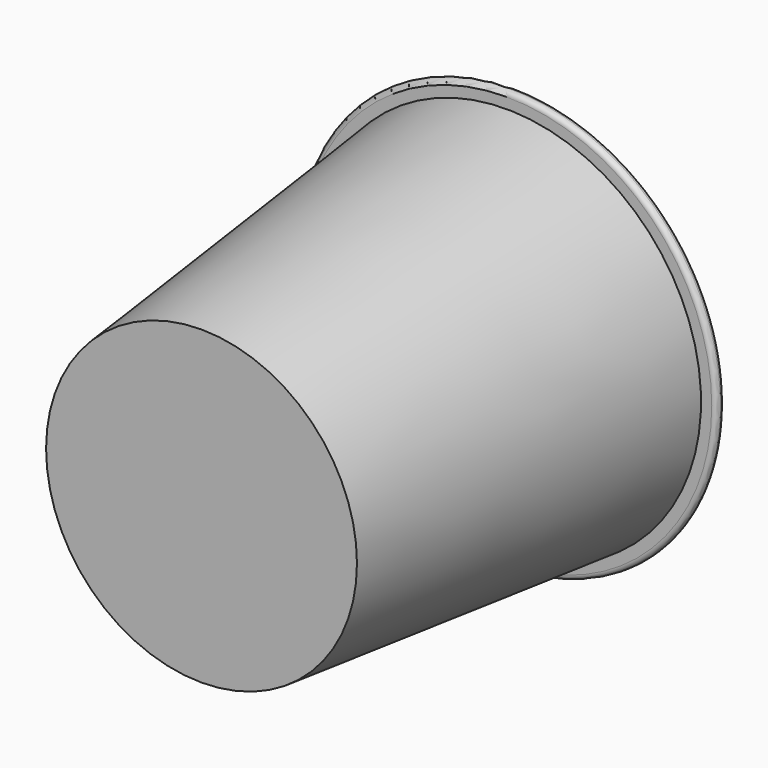
from build123d import *

# Parameters (mm, degrees)
F2_R = 0.99999
F3_R = 1


# Not quite as in the source:
# - a fillet or chamfer is up to 0.001 mm smaller than in the source, because OpenCascade refuses the exact size


with BuildPart() as f1:
    # F0 (on Top) → F1 (revolve)
    with BuildSketch(Plane.XY):
        Polygon((-31.8053636701, 0), (0, 0), (0, 2), (-30, 2), (-38, 80), (-43, 80), (-43, 78), (-39.8053636701, 78), align=None)
    revolve(axis=Axis((0, 3.6410242221, 0), (0, -1, 0)))

    # F2 (radius 1 in the source; OpenCascade refuses exactly that, so slightly less here)
    f2_edges = [f1.edges().sort_by_distance(p)[0] for p in [
        (43, 80, 0),
        (43, 78, 0),
        (-43, 79, 0),
    ]]
    fillet(f2_edges, radius=F2_R)

    # F3
    f3_edges = [f1.edges().sort_by_distance(p)[0] for p in [
        (38, 80, 0),
    ]]
    fillet(f3_edges, radius=F3_R)


solid = f1.part
